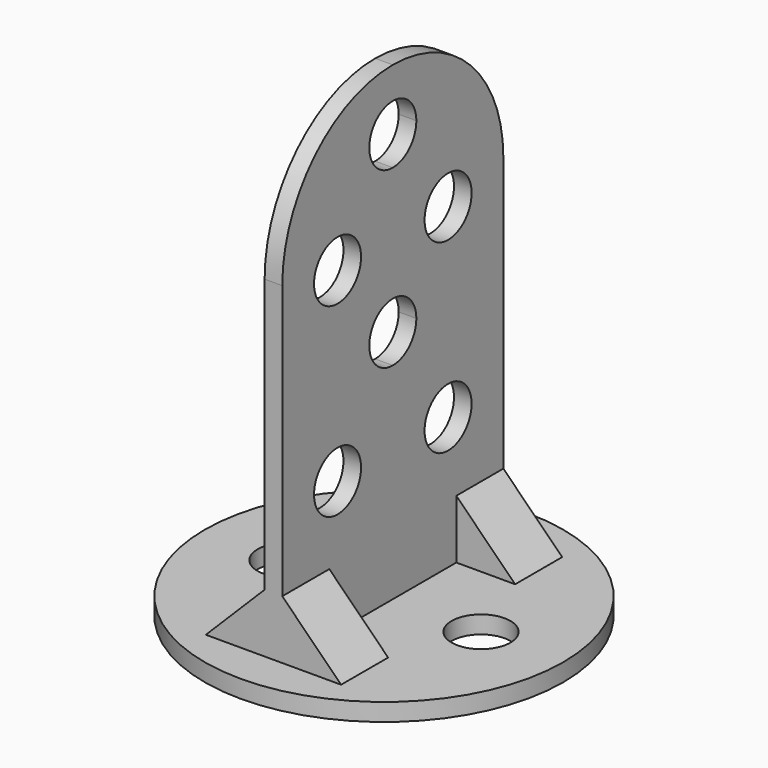
from build123d import *

# Parameters (mm, degrees)
F0_R      = 30.5
F1_DEPTH  = 3
F3_DEPTH  = 80
F4_R      = 23.49999
F5_W      = 10
F5_H      = 10
F6_DEPTH  = 10
F7_SIZE   = 9.99999
F8_W      = 10
F8_H      = 10
F9_DEPTH  = 10
F10_SIZE  = 9.99999
F11_R     = 5
F12_DEPTH = 3
F13_R     = 5
F14_DEPTH = 3


# Not quite as in the source:
# - a fillet or chamfer is up to 0.001 mm smaller than in the source, because OpenCascade refuses the exact size


with BuildPart() as f1:
    # F0 (on Top) → F1 (new body)
    with BuildSketch(Plane.XY):
        Circle(F0_R)
    extrude(amount=F1_DEPTH)

    # F2 (on face) → F3 (join)
    with BuildSketch(Plane.XY.offset(3)):
        Polygon((1.5, 23.5), (0, 23.5), (-1.5, 23.5), (-1.5, 0), (-1.5, -23.5), (0, -23.5), (1.5, -23.5), (1.5, 0), align=None)
    extrude(amount=F3_DEPTH)

    # F4 (radius 23.5 in the source; OpenCascade refuses exactly that, so slightly less here)
    f4_edges = [f1.edges().sort_by_distance(p)[0] for p in [
        (0, 23.5, 83),
        (0, -23.5, 83),
    ]]
    fillet(f4_edges, radius=F4_R)

    # F5 (on face) → F6 (join)
    with BuildSketch(Plane.XY.offset(3)):
        with Locations((6.5, -18.5)):
            Rectangle(F5_W, F5_H)
    extrude(amount=F6_DEPTH)

    # F7 (size 10 in the source; OpenCascade refuses exactly that, so slightly less here)
    f7_edges = [f1.edges().sort_by_distance(p)[0] for p in [
        (11.5, -18.5, 13),
    ]]
    chamfer(f7_edges, length=F7_SIZE)

    # F8 (on face) → F9 (join)
    with BuildSketch(Plane.XY.offset(3)):
        with Locations((6.5, 18.5)):
            Rectangle(F8_W, F8_H)
        with Locations((-6.5, 18.5)):
            Rectangle(F8_W, F8_H)
        with Locations((-6.5, -18.5)):
            Rectangle(F8_W, F8_H)
    extrude(amount=F9_DEPTH)

    # F10 (size 10 in the source; OpenCascade refuses exactly that, so slightly less here)
    f10_edges = [f1.edges().sort_by_distance(p)[0] for p in [
        (11.5, 18.5, 13),
        (-11.5, 18.5, 13),
        (-11.5, -18.5, 13),
    ]]
    chamfer(f10_edges, length=F10_SIZE)

    # F11 (on face) → F12 (cut)
    with BuildSketch(Plane.XY.offset(3)):
        with BuildLine():
            ThreePointArc((21.5, 0), (16.5, 5), (11.5, 0))
            ThreePointArc((11.5, 0), (16.5, -5), (21.5, 0))
        make_face()
        with Locations((-16.5, 0)):
            Circle(F11_R)
    extrude(amount=-F12_DEPTH, mode=Mode.SUBTRACT)

    # F13 (on face) → F14 (cut)
    with BuildSketch(Plane.YZ.offset(1.5)):
        with BuildLine():
            ThreePointArc((0, 77.6050660014), (-5, 72.6050660014), (0, 67.6050660014))
            ThreePointArc((0, 67.6050660014), (3.5355339059, 69.0695320955), (5, 72.6050660014))
            ThreePointArc((5, 72.6050660014), (3.5355339059, 76.1405999073), (0, 77.6050660014))
        make_face()
        with Locations((11.75, 57.0152029395)):
            Circle(F13_R)
        with BuildLine():
            ThreePointArc((0, 48), (-5, 43), (0, 38))
            ThreePointArc((0, 38), (3.5355339059, 39.4644660941), (5, 43))
            ThreePointArc((5, 43), (3.5355339059, 46.5355339059), (0, 48))
        make_face()
        with Locations((-11.75, 57.0152029395)):
            Circle(F13_R)
        with Locations((-11.75, 25.4681762308)):
            Circle(F13_R)
        with Locations((11.75, 25.4681762308)):
            Circle(F13_R)
    extrude(amount=-F14_DEPTH, mode=Mode.SUBTRACT)


solid = f1.part
